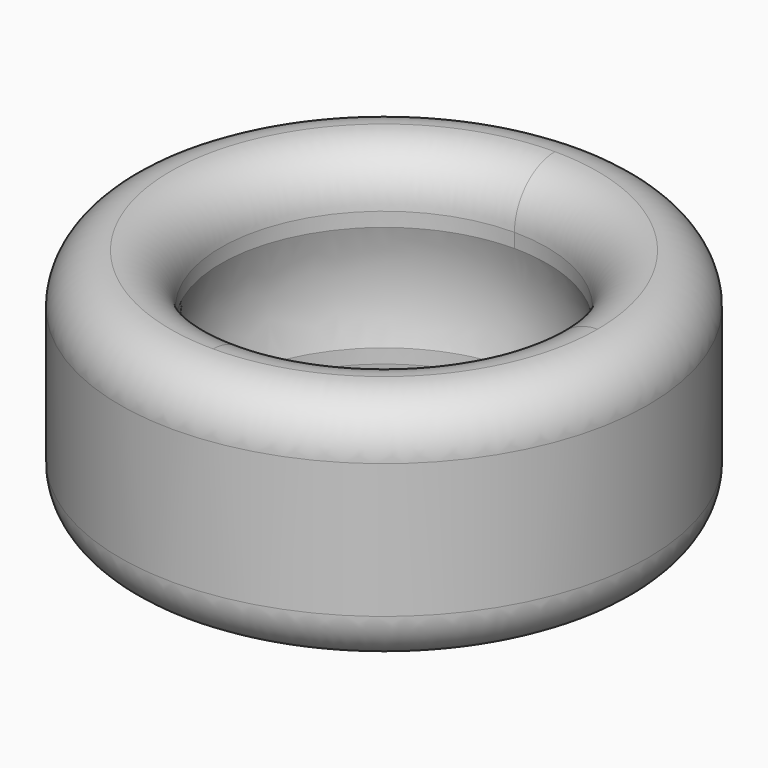
from build123d import *

# Parameters (mm, degrees)
F0_R     = 7.85
F1_DEPTH = 3.5
F3_R     = 1.49999


# Not quite as in the source:
# - a fillet or chamfer is up to 0.001 mm smaller than in the source, because OpenCascade refuses the exact size


with BuildPart() as f1:
    # F0 (on Top) → F1 (new body, symmetric)
    with BuildSketch(Plane.XY):
        Circle(F0_R)
        with BuildLine():
            ThreePointArc((0, -4.85), (-4.85, 0), (0, 4.85))
            Line((0, 4.85), (0, 5.1))
            ThreePointArc((0, 5.1), (5.1, 0), (0, -5.1))
            Line((0, -5.1), (0, -4.85))
        make_face(mode=Mode.SUBTRACT)
        with BuildLine():
            ThreePointArc((0, 4.85), (3.4294678888, 3.4294678888), (4.85, 0))
            ThreePointArc((4.85, 0), (3.4294678888, -3.4294678888), (0, -4.85))
            Line((0, -4.85), (0, -5.1))
            ThreePointArc((0, -5.1), (5.1, 0), (0, 5.1))
            Line((0, 5.1), (0, 4.85))
        make_face()
    extrude(amount=F1_DEPTH, both=True)

    # F0 (on Top) → F2 (revolve, cut)
    with BuildSketch(Plane.XY):
        with BuildLine():
            ThreePointArc((0, -4.85), (3.4294678888, -3.4294678888), (4.85, 0))
            ThreePointArc((4.85, 0), (3.4294678888, 3.4294678888), (0, 4.85))
            Line((0, 4.85), (0, -4.85))
        make_face()
        with BuildLine():
            ThreePointArc((0, 4.85), (3.4294678888, 3.4294678888), (4.85, 0))
            ThreePointArc((4.85, 0), (3.4294678888, -3.4294678888), (0, -4.85))
            Line((0, -4.85), (0, -5.1))
            ThreePointArc((0, -5.1), (5.1, 0), (0, 5.1))
            Line((0, 5.1), (0, 4.85))
        make_face()
    revolve(axis=Axis((0, 0, 0), (0, -1, 0)), mode=Mode.SUBTRACT)

    # F3 (radius 1.5 in the source; OpenCascade refuses exactly that, so slightly less here)
    f3_edges = [f1.edges().sort_by_distance(p)[0] for p in [
        (-7.85, 0, 3.5),
        (0, -4.85, 3.5),
        (0, -4.85, -3.5),
        (-7.85, 0, -3.5),
    ]]
    fillet(f3_edges, radius=F3_R)


solid = f1.part
